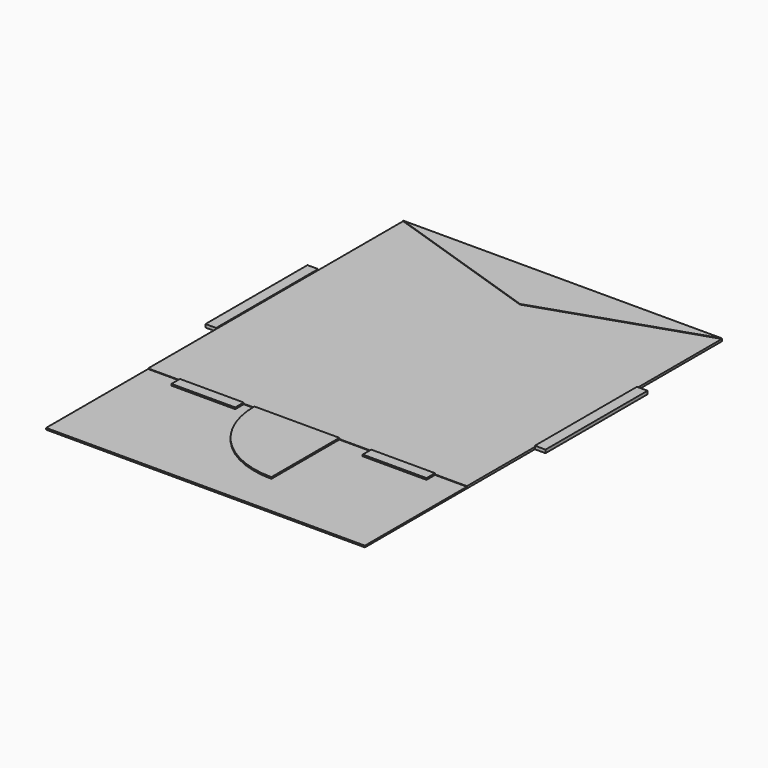
from build123d import *

# Parameters (mm, degrees)
F1_DEPTH = 25
F0_W     = 100
F0_H     = 1200
F2_DEPTH = 30
F0_W_2   = 600
F0_H_2   = 100
F3_DEPTH = 30
F4_DEPTH = 15
F5_DEPTH = 20


# Not quite as in the source:
# - a feature names something its author has since deleted; it is built from what else it names


with BuildPart() as f1:
    # F0 (on Top) → F1 (new body)
    with BuildSketch(Plane.XY):
        Polygon((3000, 4200), (0, 4200), (1500, 3700), align=None)
    extrude(amount=F1_DEPTH)



with BuildPart() as f2:
    # F0 (on Top) → F2 (new body)
    with BuildSketch(Plane.XY):
        with Locations((-50, 2600)):
            Rectangle(F0_W, F0_H)
    extrude(amount=F2_DEPTH)


with BuildPart() as f2b:
    # F0 (on Top) → F2, piece 2 (new body)
    with BuildSketch(Plane.XY):
        with Locations((3050, 2600)):
            Rectangle(F0_W, F0_H)
    extrude(amount=F2_DEPTH)


with BuildPart() as f2c:
    # F0 (on Top) → F2, piece 3 (new body)
    with BuildSketch(Plane.XY):
        with Locations((2400, 1150)):
            Rectangle(F0_W_2, F0_H_2)
    extrude(amount=F2_DEPTH)



with BuildPart() as f2d:
    # F0 (on Top) → F2, piece 4 (new body)
    with BuildSketch(Plane.XY):
        with Locations((600, 1150)):
            Rectangle(F0_W_2, F0_H_2)
    extrude(amount=F2_DEPTH)


with BuildPart() as f3:
    # F0 (on Top) → F3 (new body)
    with BuildSketch(Plane.XY):
        with BuildLine():
            Line((1800, 1200), (1000, 1200))
            ThreePointArc((1000, 1200), (1234.3145750508, 634.3145750508), (1800, 400))
            Line((1800, 400), (1800, 1200))
        make_face()
    extrude(amount=F3_DEPTH)


with BuildPart() as f2c_1:
    add(f2c.part)

    add(f2d.part)  # F4 merges F2d

    add(f3.part)  # F4 merges F3
    # F0 (on Top) → F4 (join)
    with BuildSketch(Plane.XY):
        with BuildLine():
            Line((0, 1200), (0, 0))
            Line((0, 0), (3000, 0))
            Line((3000, 0), (3000, 1200))
            Line((3000, 1200), (2700, 1200))
            Line((2700, 1200), (2700, 1100))
            Line((2700, 1100), (2100, 1100))
            Line((2100, 1100), (2100, 1200))
            Line((2100, 1200), (1800, 1200))
            Line((1800, 1200), (1800, 400))
            ThreePointArc((1800, 400), (1234.3145750508, 634.3145750508), (1000, 1200))
            Line((1000, 1200), (900, 1200))
            Line((900, 1200), (900, 1100))
            Line((900, 1100), (300, 1100))
            Line((300, 1100), (300, 1200))
            Line((300, 1200), (0, 1200))
        make_face()
    extrude(amount=F4_DEPTH)


with BuildPart() as f1_1:
    add(f1.part)

    add(f2.part)  # F5 merges F2

    add(f2b.part)  # F5 merges F2b

    add(f2c_1.part)  # F5 merges F2c
    # F0 (on Top) → F5 (join)
    with BuildSketch(Plane.XY):
        Polygon((0, 2000), (0, 1200), (300, 1200), (900, 1200), (1000, 1200), (1800, 1200), (2100, 1200), (2700, 1200), (3000, 1200), (3000, 2000), (3000, 3200), (3000, 4200), (1500, 3700), (0, 4200), (0, 3200), align=None)
    extrude(amount=F5_DEPTH)


solid = f1_1.part
